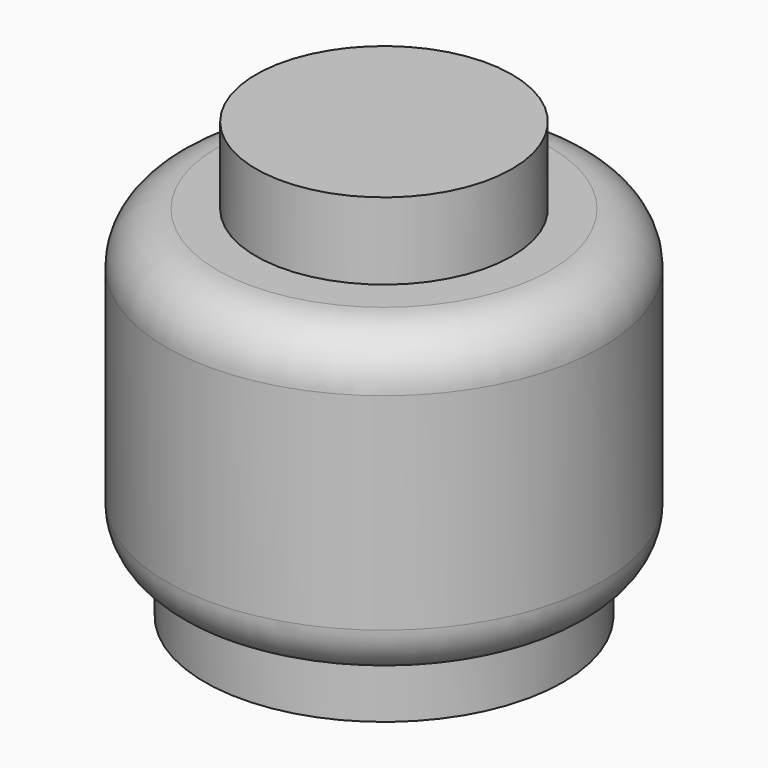
from build123d import *

# Parameters (mm, degrees)
F0_R     = 3.5
F1_DEPTH = 1
F2_R     = 4.25
F3_DEPTH = 6
F4_R     = 2.5
F5_DEPTH = 1.5
F7_R     = 2.5
F8_DEPTH = 6


# Not quite as in the source:
# - a fillet or chamfer that OpenCascade refuses, or shapes differently, is made with other operations: its cross-section is extruded or revolved along the edge and cut away or added


with BuildPart() as f1:
    # F0 (on Top) → F1 (new body)
    with BuildSketch(Plane.XY):
        Circle(F0_R)
    extrude(amount=F1_DEPTH)

    # F2 (on face) → F3 (join)
    with BuildSketch(Plane.XY.offset(1)):
        Circle(F2_R)
    extrude(amount=F3_DEPTH)

    # F4 (on face) → F5 (join)
    with BuildSketch(Plane.XY.offset(7)):
        Circle(F4_R)
    extrude(amount=F5_DEPTH)

    # F6: fillet of radius 1 on 2 edges, made by hand

    # F6_s1 → F6_t2 (revolve, cut)
    with BuildSketch(Plane.XZ):
        with BuildLine():
            ThreePointArc((4.25, 6), (3.9571067812, 6.7071067812), (3.25, 7))
            Line((3.25, 7), (4.25, 7))
            Line((4.25, 7), (4.25, 6))
        make_face()
    revolve(axis=Axis((0, 0, 7), (0, 0, 1)), mode=Mode.SUBTRACT)

    # F6_s3 → F6_t4 (revolve, cut)
    with BuildSketch(Plane.XZ):
        with BuildLine():
            ThreePointArc((4.25, 1.9682458366), (4.040569415, 1.3558734009), (3.5, 1))
            Line((3.5, 1), (4.25, 1))
            Line((4.25, 1), (4.25, 1.9682458366))
        make_face()
    revolve(axis=Axis((0, 0, 1), (0, 0, 1)), mode=Mode.SUBTRACT)

    # F7 (on face) → F8 (cut)
    with BuildSketch(Plane(origin=(0, 0, 0), x_dir=(1, 0, 0), z_dir=(0, 0, -1))):
        Circle(F7_R)
    extrude(amount=-F8_DEPTH, mode=Mode.SUBTRACT)


solid = f1.part
